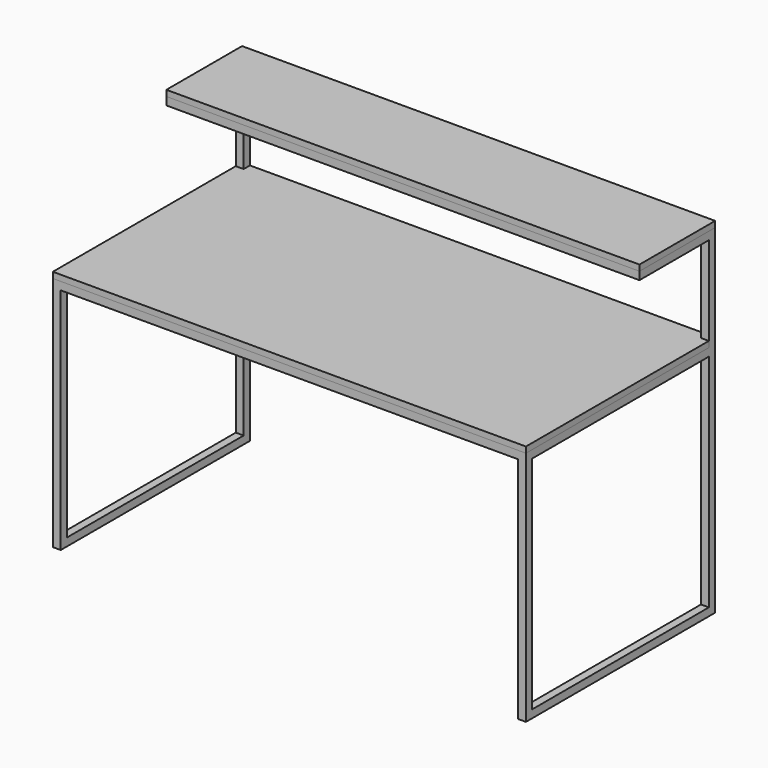
from build123d import *

# Parameters (mm, degrees)
F0_W      = 1524
F0_H      = 762
F0_W_2    = 1473.2
F0_H_2    = 711.2
F1_DEPTH  = 25.4
F2_W      = 25.4
F2_H      = 25.4
F3_DEPTH  = 736.6
F4_W      = 25.4
F4_H      = 25.4
F5_DEPTH  = 304.8
F6_W      = 1524
F6_H      = 304.8
F6_W_2    = 1473.2
F6_H_2    = 254
F7_DEPTH  = 25.4
F8_W      = 711.2
F8_H      = 25.4
F9_DEPTH  = 25.4
F10_W     = 711.2
F10_H     = 25.4
F11_DEPTH = 25.4
F13_DEPTH = 19.05
F14_W     = 1524
F14_H     = 304.8
F14_W_2   = 1473.2
F14_H_2   = 254
F15_DEPTH = 19.05


# Not quite as in the source:
# - a length typed as a fraction of an inch, garbled in the dataset ("3 / 203.2 mm" for 3/8 in), is restored
# - a feature names something its author has since deleted; it is built from what else it names


with BuildPart() as f1:
    # F0 (on Top) → F1 (new body)
    with BuildSketch(Plane.XY):
        Rectangle(F0_W, F0_H)
        Rectangle(F0_W_2, F0_H_2, mode=Mode.SUBTRACT)
    extrude(amount=F1_DEPTH)

    # F2 (on face) → F3 (join)
    with BuildSketch(Plane(origin=(0, 0, 0), x_dir=(1, 0, 0), z_dir=(0, 0, -1))):
        with Locations((-749.3, 368.3)):
            Rectangle(F2_W, F2_H)
        with Locations((-749.3, -368.3)):
            Rectangle(F2_W, F2_H)
        with Locations((749.3, -368.3)):
            Rectangle(F2_W, F2_H)
        with Locations((749.3, 368.3)):
            Rectangle(F2_W, F2_H)
    extrude(amount=F3_DEPTH)

    # F4 (on face) → F5 (join)
    with BuildSketch(Plane.XY.offset(25.4)):
        with Locations((749.3, 368.3)):
            Rectangle(F4_W, F4_H)
        with Locations((-749.3, 368.3)):
            Rectangle(F4_W, F4_H)
    extrude(amount=F5_DEPTH)

    # F6 (on face) → F7 (join)
    with BuildSketch(Plane.XY.offset(330.2)):
        with Locations((0, 228.6)):
            Rectangle(F6_W, F6_H)
        with Locations((0, 228.6)):
            Rectangle(F6_W_2, F6_H_2, mode=Mode.SUBTRACT)
    extrude(amount=F7_DEPTH)

    # F8 (on face) → F9 (join)
    with BuildSketch(Plane.YZ.offset(762)):
        with Locations((0, -723.9)):
            Rectangle(F8_W, F8_H)
    extrude(amount=-F9_DEPTH)

    # F10 (on face) → F11 (join)
    with BuildSketch(Plane(origin=(-762, 0, 0), x_dir=(0, -1, 0), z_dir=(-1, 0, 0))):
        with Locations((0, -723.9)):
            Rectangle(F10_W, F10_H)
    extrude(amount=-F11_DEPTH)


with BuildPart() as f13:
    # F12 (on face) → F13 (new body)
    with BuildSketch(Plane.XY.offset(25.4)):
        Polygon((-736.6, 381), (-736.6, 355.6), (-736.6, -355.6), (736.6, -355.6), (736.6, 355.6), (736.6, 381), align=None)
        Polygon((-762, 355.6), (-762, -381), (762, -381), (762, 355.6), (736.6, 355.6), (736.6, -355.6), (-736.6, -355.6), (-736.6, 355.6), align=None)
    extrude(amount=F13_DEPTH)


with BuildPart() as f15:
    # F14 (on face) → F15 (new body)
    with BuildSketch(Plane.XY.offset(355.6)):
        with Locations((0, 228.6)):
            Rectangle(F14_W, F14_H)
        with Locations((0, 228.6)):
            Rectangle(F14_W_2, F14_H_2, mode=Mode.SUBTRACT)
        with Locations((0, 228.6)):
            Rectangle(F14_W_2, F14_H_2)
    extrude(amount=F15_DEPTH)


solid = Compound([f1.part, f13.part, f15.part])
